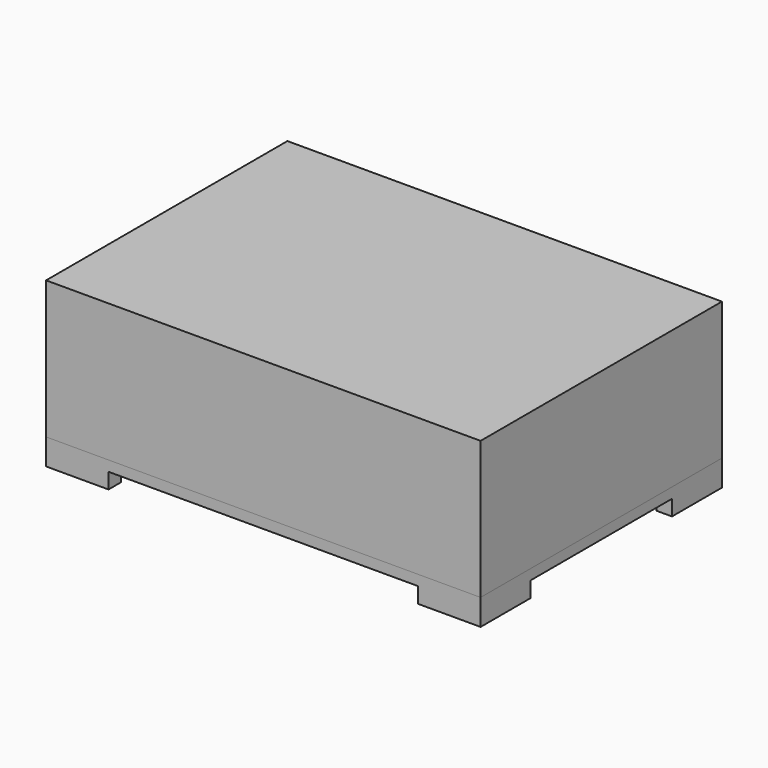
from build123d import *

# Parameters (mm, degrees)
F0_W      = 77.5417897031
F0_H      = 52
F0_W_2    = 22.5
F0_H_2    = 22.5
F1_DEPTH  = 10
F2_W      = 81.5417897031
F2_H      = 56
F3_DEPTH  = 3
F4_W      = 83.5417897031
F4_H      = 58
F5_DEPTH  = 2
F6_SIZE   = 1
F7_SIZE   = 0.99999
F9_DEPTH  = 3
F10_W     = 83.5417897031
F10_H     = 58
F10_W_2   = 81.5417897031
F10_H_2   = 56
F11_DEPTH = 25.5
F12_W     = 83.5417897031
F12_H     = 58
F13_DEPTH = 1


# Not quite as in the source:
# - a fillet or chamfer is up to 0.001 mm smaller than in the source, because OpenCascade refuses the exact size


with BuildPart() as f1:
    # F0 (on Top) → F1 (new body)
    with BuildSketch(Plane.XY):
        with Locations((36.7291051485, 24)):
            Rectangle(F0_W, F0_H)
        with Locations((11.25, 11.25)):
            Rectangle(F0_W_2, F0_H_2, mode=Mode.SUBTRACT)
        with Locations((36.75, 11.25)):
            Rectangle(F0_W_2, F0_H_2, mode=Mode.SUBTRACT)
        with Locations((62.25, 11.25)):
            Rectangle(F0_W_2, F0_H_2, mode=Mode.SUBTRACT)
        with Locations((11.25, 36.75)):
            Rectangle(F0_W_2, F0_H_2, mode=Mode.SUBTRACT)
        with Locations((36.75, 36.75)):
            Rectangle(F0_W_2, F0_H_2, mode=Mode.SUBTRACT)
        with Locations((62.25, 36.75)):
            Rectangle(F0_W_2, F0_H_2, mode=Mode.SUBTRACT)
    extrude(amount=F1_DEPTH)

    # F2 (on face) → F3 (join)
    with BuildSketch(Plane(origin=(0, 0, 0), x_dir=(1, 0, 0), z_dir=(0, 0, -1))):
        with Locations((36.7291051485, -24)):
            Rectangle(F2_W, F2_H)
    extrude(amount=F3_DEPTH)

    # F4 (on face) → F5 (join)
    with BuildSketch(Plane(origin=(0, 0, -3), x_dir=(1, 0, 0), z_dir=(0, 0, -1))):
        with Locations((36.7291051485, -24)):
            Rectangle(F4_W, F4_H)
    extrude(amount=F5_DEPTH)

    # F6
    f6_edges = [f1.edges().sort_by_distance(p)[0] for p in [
        (77.5, 24, 0),
        (36.729105, 52, 0),
        (-4.04179, 24, 0),
        (36.729105, -4, 0),
    ]]
    chamfer(f6_edges, length=F6_SIZE)

    # F7 (size 1 in the source; OpenCascade refuses exactly that, so slightly less here)
    f7_edges = [f1.edges().sort_by_distance(p)[0] for p in [
        (22.5, 11.25, 10),
        (11.25, 0, 10),
        (0, 11.25, 10),
        (11.25, 22.5, 10),
        (48, 11.25, 10),
        (36.75, 0, 10),
        (25.5, 11.25, 10),
        (36.75, 22.5, 10),
        (62.25, 22.5, 10),
        (73.5, 11.25, 10),
        (62.25, 0, 10),
        (51, 11.25, 10),
        (62.25, 25.5, 10),
        (73.5, 36.75, 10),
        (62.25, 48, 10),
        (51, 36.75, 10),
        (36.75, 25.5, 10),
        (48, 36.75, 10),
        (36.75, 48, 10),
        (22.5, 36.75, 10),
        (11.25, 25.5, 10),
        (0, 36.75, 10),
        (-2.04179, 24, 10),
        (36.729105, -2, 10),
        (75.5, 24, 10),
        (36.729105, 50, 10),
        (11.25, 48, 10),
        (25.5, 36.75, 10),
        (36.729105, 50, 0),
        (-2.04179, 24, 0),
        (75.5, 24, 0),
        (36.729105, -2, 0),
        (-4.04179, -4, -2),
        (-4.04179, 52, -2),
        (77.5, 52, -2),
        (77.5, -4, -2),
    ]]
    chamfer(f7_edges, length=F7_SIZE)

    # F8 (on face) → F9 (join)
    with BuildSketch(Plane(origin=(0, 0, -5), x_dir=(1, 0, 0), z_dir=(0, 0, -1))):
        Polygon((75.5, -7), (78.5, -7), (78.5, 5), (66.5, 5), (66.5, 2), (75.5, 2), align=None)
        Polygon((66.5, -53), (78.5, -53), (78.5, -41), (75.5, -41), (75.5, -50), (66.5, -50), align=None)
        Polygon((-5.0417897031, -53), (6.9582102969, -53), (6.9582102969, -50), (-2.0417897031, -50), (-2.0417897031, -41), (-5.0417897031, -41), align=None)
        Polygon((6.9582102969, 2), (6.9582102969, 5), (-5.0417897031, 5), (-5.0417897031, -7), (-2.0417897031, -7), (-2.0417897031, 2), align=None)
    extrude(amount=F9_DEPTH)


with BuildPart() as f11:
    # F10 (on face) → F11 (new body)
    with BuildSketch(Plane.XY.offset(-3)):
        with Locations((36.7291051485, 24)):
            Rectangle(F10_W, F10_H)
        with Locations((36.7291051485, 24)):
            Rectangle(F10_W_2, F10_H_2, mode=Mode.SUBTRACT)
    extrude(amount=F11_DEPTH)

    # F12 (on face) → F13 (join)
    with BuildSketch(Plane.XY.offset(22.5)):
        with Locations((36.7291051485, 24)):
            Rectangle(F12_W, F12_H)
    extrude(amount=F13_DEPTH)


solid = Compound([f1.part, f11.part])
